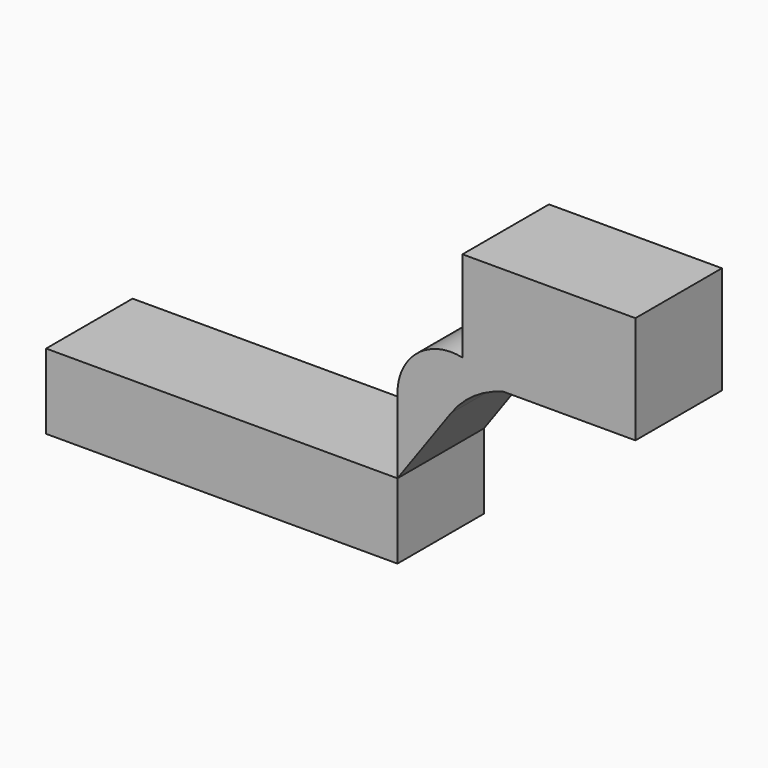
from build123d import *

# Parameters (mm, degrees)
F0_W     = 20.3160279515
F0_H     = 3.888219498
F1_DEPTH = 12.7
F0_W_2   = 82.55
F0_H_2   = 17.6465612206


with BuildPart() as f1:
    # F0 (on Front) → F1 (new body, symmetric)
    with BuildSketch(Plane.XZ):
        with BuildLine():
            Line((41.275, 26.4365587761), (41.275, 8.8232806103))
            Line((41.275, 8.8232806103), (53.8858462351, 26.4365587761))
            ThreePointArc((53.8858462351, 26.4365587761), (59.3031752306, 31.7323772422), (66.2102704506, 34.8444797939))
            Line((66.2102704506, 34.8444797939), (56.5511865373, 34.8444797939))
            Line((56.5511865373, 34.8444797939), (56.5511865373, 38.7625233971))
            ThreePointArc((56.5511865373, 38.7625233971), (45.9668423189, 36.2509777472), (41.275, 26.4365587761))
        make_face()
        with BuildLine():
            ThreePointArc((56.6855553593, 38.7326992919), (56.6184116374, 38.747794664), (56.5511865373, 38.7625233971))
            Line((56.5511865373, 38.7625233971), (56.5511865373, 34.8444797939))
            Line((56.5511865373, 34.8444797939), (66.2102704506, 34.8444797939))
            ThreePointArc((66.2102704506, 34.8444797939), (71.5387424697, 35.508505706), (76.8672144887, 34.8444797939))
            Line((76.8672144887, 34.8444797939), (76.8672144887, 38.7326992919))
            Line((76.8672144887, 38.7326992919), (56.6855553593, 38.7326992919))
        make_face()
        with BuildLine():
            Line((56.5511865373, 60.1290911436), (56.5511865373, 38.7625233971))
            ThreePointArc((56.5511865373, 38.7625233971), (56.6184116374, 38.747794664), (56.6855553593, 38.7326992919))
            Line((56.6855553593, 38.7326992919), (56.6855553593, 60.1290911436))
            Line((56.6855553593, 60.1290911436), (56.5511865373, 60.1290911436))
        make_face()
        with BuildLine():
            ThreePointArc((76.8672144887, 34.8444797939), (71.5387424697, 35.508505706), (66.2102704506, 34.8444797939))
            Line((66.2102704506, 34.8444797939), (76.8672144887, 34.8444797939))
        make_face()
        Polygon((56.6855553593, 60.1290911436), (56.6855553593, 38.7326992919), (76.8672144887, 38.7326992919), (97.1832424402, 38.7326992919), (97.1832424402, 60.1290911436), align=None)
        with Locations((87.0252284645, 36.7885895429)):
            Rectangle(F0_W, F0_H)
    extrude(amount=F1_DEPTH, both=True)


with BuildPart() as f1b:
    # F0 (on Front) → F1, piece 2 (new body, symmetric)
    with BuildSketch(Plane.XZ):
        Rectangle(F0_W_2, F0_H_2)
    extrude(amount=F1_DEPTH, both=True)


solid = Compound([f1.part, f1b.part])
